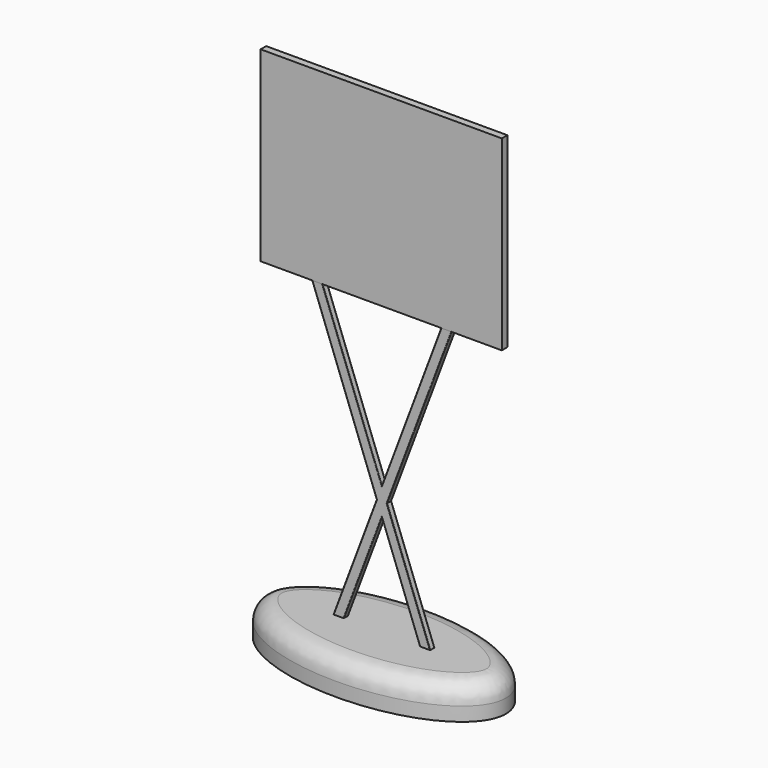
from build123d import *

# Parameters (mm, degrees)
F2_DEPTH      = 12
F1_W          = 86.7539048195
F1_H          = 67.1276152134
F3_DEPTH      = 1.25
F3_DEPTH_BACK = 1.25
F5_DEPTH      = 1
F5_DEPTH_BACK = 1
F6_R          = 7
F7_R          = 0.2


with BuildPart() as f2:
    # F0 (on Top) → F2 (new body)
    with BuildSketch(Plane.XY):
        with BuildLine():
            add(Edge.make_bspline(
                [(43.8235126286, 0), (43.8235126286, 37.7366478253), (-21.9117563143, 18.8683239126), (-87.6470252571, 0), (-21.9117563143, -18.8683239126), (43.8235126286, -37.7366478253), (43.8235126286, 0)],
                knots=[0, 0, 0, 2.0943951024, 2.0943951024, 4.1887902048, 4.1887902048, 6.2831853072, 6.2831853072, 6.2831853072], degree=2, weights=[1, 0.5, 1, 0.5, 1, 0.5, 1]))
        make_face()
    extrude(amount=F2_DEPTH)

    # F6
    f6_edges = [f2.edges().sort_by_distance(p)[0] for p in [
        (-43.823513, 6e-06, 12),
    ]]
    fillet(f6_edges, radius=F6_R)


with BuildPart() as f3:
    # F1 (on Front) → F3 (new body, two sides)
    with BuildSketch(Plane.XZ) as f3_sk:
        with Locations((0, 149.0442156792)):
            Rectangle(F1_W, F1_H)
    extrude(amount=F3_DEPTH)
    extrude(f3_sk.sketch, amount=-F3_DEPTH_BACK)


with BuildPart() as f5:
    # F4 (on Front) → F5 (new body, two sides)
    with BuildSketch(Plane.XZ) as f5_sk:
        Polygon((-17.833967352, 10.8678905179), (-14.5570435037, 9.6383499157), (0, 48.4352167556), (-1.8691310154, 53.4167521266), align=None)
        Polygon((-1.8691310154, 53.4167521266), (0, 48.4352167556), (1.8691310154, 53.4167521266), (0, 58.3982874977), align=None)
        Polygon((1.8691310154, 53.4167521266), (0, 48.4352167556), (14.5570435037, 9.6383499157), (17.833967352, 10.8678905179), align=None)
        Polygon((0, 58.3982874977), (1.8691310154, 53.4167521266), (26.9801891933, 120.3417688783), (23.703265345, 121.5713094805), align=None)
        Polygon((-26.9801891933, 120.3417688783), (-1.8691310154, 53.4167521266), (0, 58.3982874977), (-23.703265345, 121.5713094805), align=None)
    extrude(amount=F5_DEPTH)
    extrude(f5_sk.sketch, amount=-F5_DEPTH_BACK)

    # F7
    f7_edges = [f5.edges().sort_by_distance(p)[0] for p in [
        (-11.851633, -1, 89.984798),
        (-11.851633, 1, 89.984798),
        (14.42466, -1, 86.879261),
        (11.851633, -1, 89.984798),
        (14.42466, 1, 86.879261),
        (9.851549, -1, 32.142321),
        (9.851549, 1, 32.142321),
        (-7.278522, -1, 29.036783),
        (-7.278522, 1, 29.036783),
        (-9.851549, -1, 32.142321),
        (-14.42466, -1, 86.879261),
        (-9.851549, 1, 32.142321),
        (-14.42466, 1, 86.879261),
        (7.278522, 1, 29.036783),
        (7.278522, -1, 29.036783),
    ]]
    fillet(f7_edges, radius=F7_R)


solid = Compound([f2.part, f3.part, f5.part])
